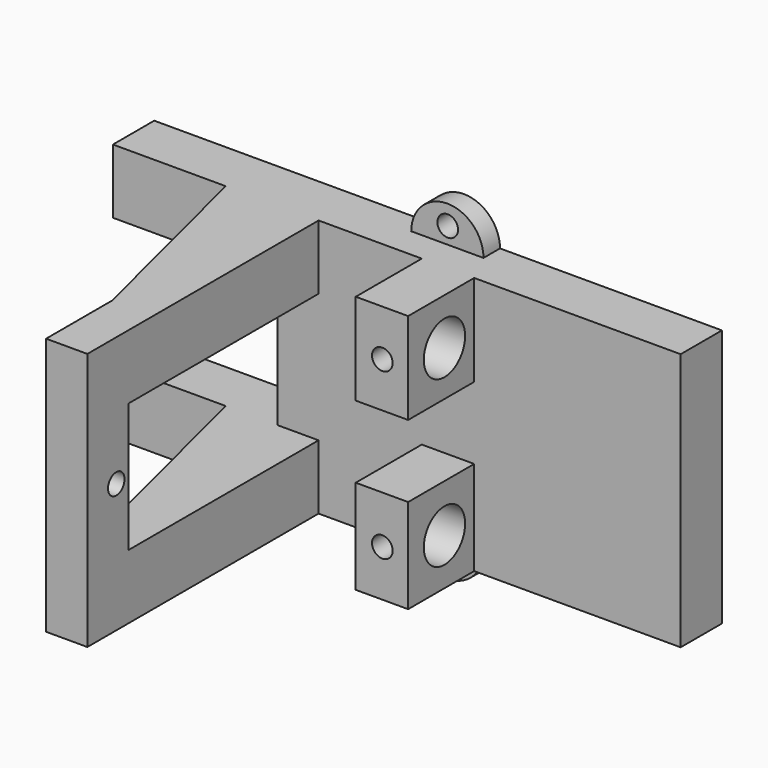
from build123d import *

# Parameters (mm, degrees)
F0_W          = 55
F0_H          = 25
F1_DEPTH      = 5
F2_W          = 15.9233940393
F2_H          = 12.5
F3_DEPTH      = 5.001
F4_R          = 1
F5_DEPTH      = 3.5
F7_DEPTH      = 28
F8_W          = 23
F8_H          = 12.5
F9_DEPTH      = 39.0776059607
F10_R         = 1
F11_DEPTH     = 39.0776059607
F12_W         = 5.0766059607
F12_H         = 8.8610539977
F12_H_2       = 9.1389460023
F13_DEPTH     = 8
F14_R         = 2.5
F15_DEPTH     = 10
F16_T1_DEPTH  = 6.25
F16_T3_DEPTH  = 6.25
F16_T8_DEPTH  = 58.1925499954
F16_T14_DEPTH = 58.1925499954
F17_R         = 1
F18_DEPTH     = 3
F20_DEPTH     = 2
F21_R         = 1
F22_DEPTH     = 2.001


# Not quite as in the source:
# - a fillet or chamfer that OpenCascade refuses, or shapes differently, is made with other operations: its cross-section is extruded or revolved along the edge and cut away or added


with BuildPart() as f1:
    # F0 (on Front) → F1 (new body)
    with BuildSketch(Plane.XZ):
        Rectangle(F0_W, F0_H)
    extrude(amount=F1_DEPTH)

    # F2 (on face) → F3 (cut, through all)
    with BuildSketch(Plane.XZ.offset(5)):
        with Locations((-19.5383029804, 0)):
            Rectangle(F2_W, F2_H)
    extrude(amount=-F3_DEPTH, mode=Mode.SUBTRACT)

    # F4 (on face) → F5 (cut)
    with BuildSketch(Plane(origin=(-11.5766059607, 0, 0), x_dir=(0, -1, 0), z_dir=(-1, 0, 0))):
        with Locations((2.5, 0)):
            Circle(F4_R)
    extrude(amount=-F5_DEPTH, mode=Mode.SUBTRACT)

    # F6 (on face) → F7 (join)
    with BuildSketch(Plane.XZ.offset(5)):
        Polygon((-7.5766059607, 12.5), (-11.5766059607, 12.5), (-11.5766059607, 6.25), (-11.5766059607, -6.25), (-11.5766059607, -12.5), (-7.5766059607, -12.5), align=None)
    extrude(amount=F7_DEPTH)

    # F8 (on face) → F9 (cut, through all)
    with BuildSketch(Plane(origin=(-11.5766059607, 0, 0), x_dir=(0, -1, 0), z_dir=(-1, 0, 0))):
        with Locations((16.5, 0)):
            Rectangle(F8_W, F8_H)
    extrude(amount=-F9_DEPTH, mode=Mode.SUBTRACT)

    # F10 (on face) → F11 (cut, through all)
    with BuildSketch(Plane(origin=(-11.5766059607, 0, 0), x_dir=(0, -1, 0), z_dir=(-1, 0, 0))):
        with Locations((29.5, 0)):
            Circle(F10_R)
    extrude(amount=-F11_DEPTH, mode=Mode.SUBTRACT)

    # F12 (on face) → F13 (join)
    with BuildSketch(Plane.XZ.offset(5)):
        with Locations((4.9616970196, 8.0694730012)):
            Rectangle(F12_W, F12_H)
        with Locations((4.9616970196, -7.9305269988)):
            Rectangle(F12_W, F12_H_2)
    extrude(amount=F13_DEPTH)

    # F14 (on face) → F15 (cut)
    with BuildSketch(Plane.YZ.offset(7.5)):
        with Locations((-8.6, 8)):
            Circle(F14_R)
        with Locations((-8.6, -8)):
            Circle(F14_R)
    extrude(amount=-F15_DEPTH, mode=Mode.SUBTRACT)

    # F16: chamfer of 20 x 5 on 2 edges, made by hand

    # F16_s2 → F16_t1 (join)
    with BuildSketch(Plane.XY.offset(6.25)):
        Polygon((-11.5766059607, -25), (-16.5766059607, -5), (-11.5766059607, -5), align=None)
    extrude(amount=F16_T1_DEPTH)

    # F16_s4 → F16_t3 (join)
    with BuildSketch(Plane.XY.offset(-12.5)):
        Polygon((-11.5766059607, -25), (-16.5766059607, -5), (-11.5766059607, -5), align=None)
    extrude(amount=F16_T3_DEPTH)


with BuildPart() as f16_tool6:
    # F16_s7 → F16_t8 (new body)
    with BuildSketch(Plane.XY.offset(12.5)):
        Polygon((-11.5766059607, -25), (-16.5766059607, -5), (-11.5766059607, -5), align=None)
    extrude(amount=-F16_T8_DEPTH)

    split(bisect_by=Plane.XY.offset(-6.25), keep=Keep.BOTTOM)

    split(bisect_by=Plane.XY.offset(-12.5), keep=Keep.TOP)


with BuildPart() as f1_1:
    add(f1.part)

    # F16_t5: union F16_tool6
    add(f16_tool6.part)


with BuildPart() as f16_tool12:
    # F16_s13 → F16_t14 (new body)
    with BuildSketch(Plane.XY.offset(45.6925499954)):
        Polygon((-11.5766059607, -25), (-16.5766059607, -5), (-11.5766059607, -5), align=None)
    extrude(amount=-F16_T14_DEPTH)

    split(bisect_by=Plane.XY.offset(12.5), keep=Keep.BOTTOM)

    split(bisect_by=Plane.XY.offset(6.25), keep=Keep.TOP)


with BuildPart() as f1_2:
    add(f1_1.part)

    # F16_t11: union F16_tool12
    add(f16_tool12.part)

    # F17 (on face) → F18 (cut)
    with BuildSketch(Plane.XZ.offset(13)):
        with Locations((5, 8)):
            Circle(F17_R)
        with Locations((5, -8)):
            Circle(F17_R)
    extrude(amount=-F18_DEPTH, mode=Mode.SUBTRACT)

    # F19 (on face) → F20 (join)
    with BuildSketch(Plane(origin=(0, 0, 0), x_dir=(-1, 0, 0), z_dir=(0, 1, 0))):
        with BuildLine():
            Line((1, -12.5), (-6, -12.5))
            ThreePointArc((-6, -12.5), (-2.5, -16), (1, -12.5))
        make_face()
        with BuildLine():
            Line((-6, 12.5), (1, 12.5))
            ThreePointArc((1, 12.5), (-2.5, 16), (-6, 12.5))
        make_face()
    extrude(amount=-F20_DEPTH)

    # F21 (on face) → F22 (cut, through all)
    with BuildSketch(Plane.XZ.offset(2)):
        with Locations((2.5334937964, 14.1)):
            Circle(F21_R)
        with Locations((2.5334937964, -14.1)):
            Circle(F21_R)
    extrude(amount=-F22_DEPTH, mode=Mode.SUBTRACT)


solid = f1_2.part
